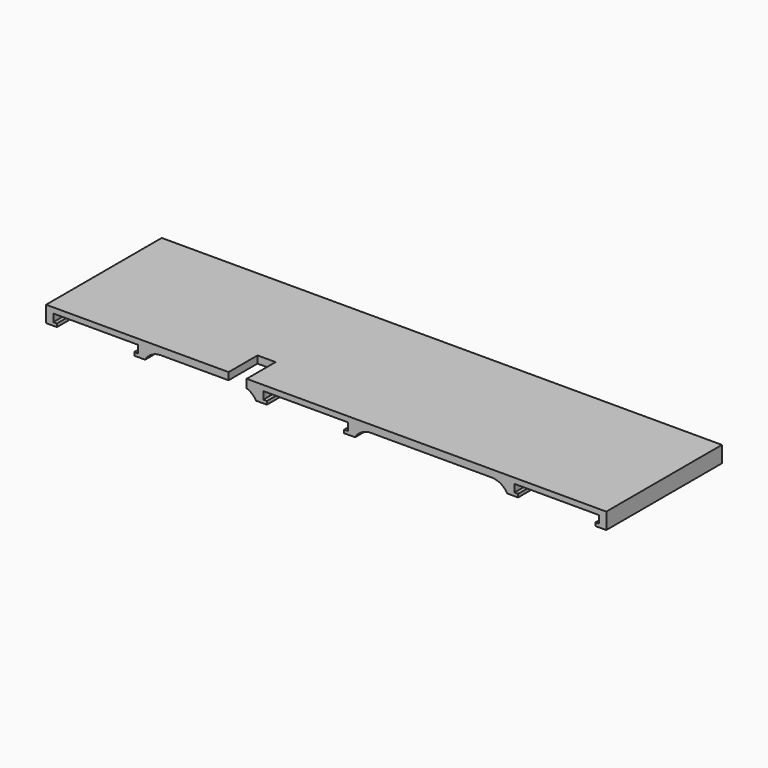
from build123d import *

# Parameters (mm, degrees)
F1_DEPTH       = 40
F2_T1_DEPTH    = 40
F5_DEPTH       = 40
F6_W           = 23.4
F6_H           = 0.5
F7_DEPTH       = 40.001
F8_T1_DEPTH    = 40
F9_W           = 5
F9_H           = 10
F10_DEPTH      = 181
F10_DEPTH_BACK = 4.501


# Not quite as in the source:
# - a fillet or chamfer that OpenCascade refuses, or shapes differently, is made with other operations: its cross-section is extruded or revolved along the edge and cut away or added
# - an extrude ends at something that could not be found from the text; its depth is read off the source's solid


with BuildPart() as f1:
    # F0 (on Front) → F1 (new body)
    with BuildSketch(Plane.XZ):
        Polygon((77.5, 0), (0, 0), (0, -2), (50.1, -2), (50.1, -4.5), (53.1, -4.5), (53.1, -3.6), (52.1, -3.6), (52.1, -2), (52.1, -1.5), (75.5, -1.5), (75.5, -2), (75.5, -3.6), (74.5, -3.6), (74.5, -4.5), (77.5, -4.5), (77.5, -2), align=None)
    extrude(amount=F1_DEPTH)

    # F2: fillet of radius 5 on 1 edges, made by hand

    # F2_s2 → F2_t1 (join)
    with BuildSketch(Plane.XZ):
        with BuildLine():
            ThreePointArc((50.1, -4.5), (48.2698729811, -2.6698729811), (45.7698729811, -2))
            Line((45.7698729811, -2), (50.1, -2))
            Line((50.1, -2), (50.1, -4.5))
        make_face()
    extrude(amount=F2_T1_DEPTH)

    # F3: F1 across plane


with BuildPart() as f1_1:
    add(f1.part)
    add(f1.part.mirror(Plane.YZ))

    # F4 (on face) → F5 (join, through all)
    with BuildSketch(Plane.XZ.offset(40)):
        Polygon((-17.4, -3.6), (-17.4, -2), (-19.4, -2), (-19.4, -4.5), (-17.4, -4.5), (-16.4, -4.5), (-16.4, -3.6), align=None)
        Polygon((8, -2), (6, -2), (6, -3.6), (5, -3.6), (5, -4.5), (6, -4.5), (8, -4.5), align=None)
    extrude(amount=-F5_DEPTH)

    # F6 (on face) → F7 (cut, through all)
    with BuildSketch(Plane(origin=(0, 0, 0), x_dir=(-1, 0, 0), z_dir=(0, 1, 0))):
        with Locations((5.7, -1.75)):
            Rectangle(F6_W, F6_H)
    extrude(amount=-F7_DEPTH, mode=Mode.SUBTRACT)

    # F8: fillet of radius 5 on 2 edges, made by hand

    # F8_s2 → F8_t1 (join)
    with BuildSketch(Plane.XZ):
        with BuildLine():
            ThreePointArc((-19.4, -4.5), (-21.2301270189, -2.6698729811), (-23.7301270189, -2))
            Line((-23.7301270189, -2), (-19.4, -2))
            Line((-19.4, -2), (-19.4, -4.5))
        make_face()
        with BuildLine():
            ThreePointArc((12.3301270189, -2), (9.8301270189, -2.6698729811), (8, -4.5))
            Line((8, -4.5), (8, -2))
            Line((8, -2), (12.3301270189, -2))
        make_face()
    extrude(amount=F8_T1_DEPTH)

    # F9 (on Top) → F10 (cut, two sides)
    with BuildSketch(Plane.XY) as f10_sk:
        with Locations((-24.5, -35)):
            Rectangle(F9_W, F9_H)
    extrude(amount=F10_DEPTH, mode=Mode.SUBTRACT)
    extrude(f10_sk.sketch, amount=-F10_DEPTH_BACK, mode=Mode.SUBTRACT)


solid = f1_1.part
